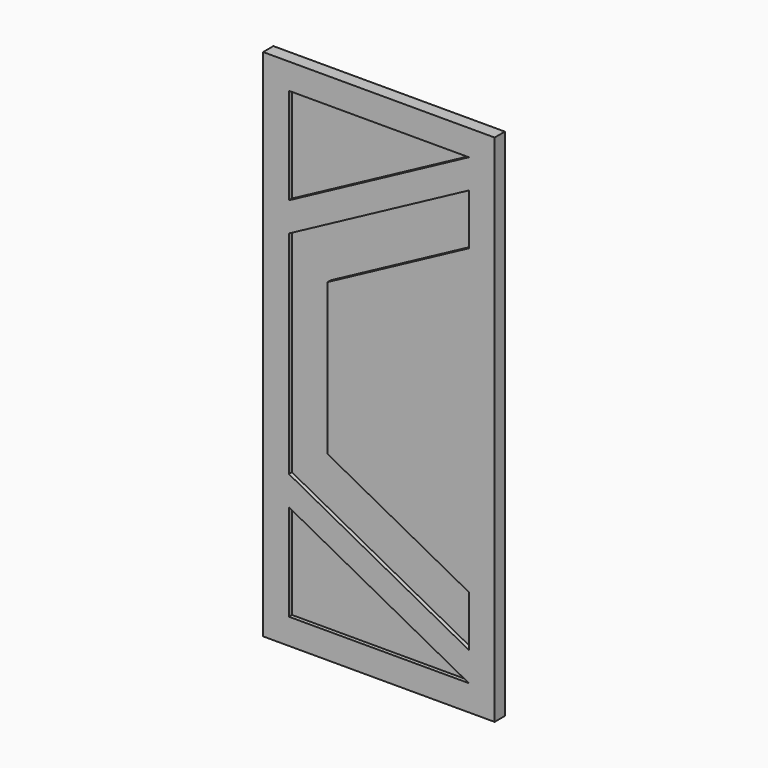
from build123d import *

# Parameters (mm, degrees)
F0_W     = 914.4
F0_H     = 2032
F1_DEPTH = 50.8
F2_W     = 152.4
F2_H     = 433.7214036722
F3_DEPTH = 15.24


with BuildPart() as f1:
    # F0 (on Front) → F1 (new body)
    with BuildSketch(Plane.XZ):
        with Locations((457.2, 1016)):
            Rectangle(F0_W, F0_H)
    extrude(amount=F1_DEPTH)

    # F2 (on face) → F3 (cut)
    with BuildSketch(Plane.XZ.offset(50.8)):
        Polygon((812.8, 1815.1392981639), (101.6, 1434.1392981639), (101.6, 1232.8607018361), (254, 1232.8607018361), (254, 1314.503558979), (812.8, 1613.8607018361), align=None)
        with Locations((177.8, 1016)):
            Rectangle(F2_W, F2_H)
        Polygon((812.8, 1930.4), (101.6, 1930.4), (101.6, 1549.4), align=None)
        Polygon((254, 799.1392981639), (101.6, 799.1392981639), (101.6, 597.8607018361), (812.8, 216.8607018361), (812.8, 418.1392981639), (254, 717.496441021), align=None)
        Polygon((101.6, 101.6), (812.8, 101.6), (101.6, 482.6), align=None)
    extrude(amount=-F3_DEPTH, mode=Mode.SUBTRACT)


solid = f1.part
